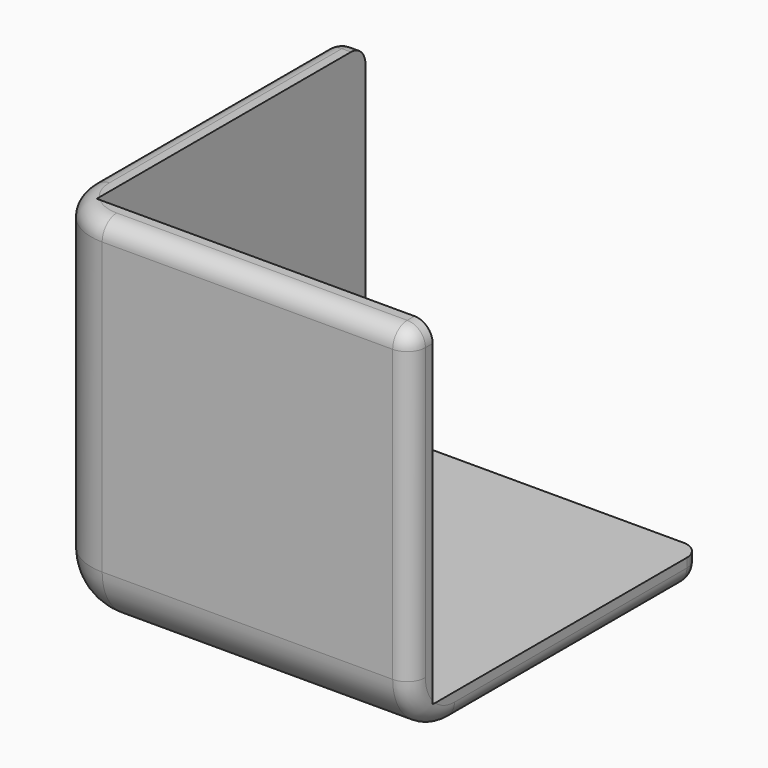
from build123d import *

# Parameters (mm, degrees)
F1_DEPTH     = 20
F3_DEPTH     = 20
F4_R         = 3
F5_T1_DEPTH  = 16
F5_T3_DEPTH  = 16
F5_T5_DEPTH  = 3
F5_T7_DEPTH  = 3
F5_T9_DEPTH  = 3
F5_T11_DEPTH = 16
F5_S15_W     = 1
F5_S15_H     = 1
F5_T16_DEPTH = 1
F5_S21_W     = 1
F5_S21_H     = 1
F5_T22_DEPTH = 1
F5_S27_W     = 1
F5_S27_H     = 1
F5_T28_DEPTH = 1
F5_T32_ANGLE = 90
F5_T34_ANGLE = 90
F5_T36_ANGLE = 90


# Not quite as in the source:
# - a fillet or chamfer that OpenCascade refuses, or shapes differently, is made with other operations: its cross-section is extruded or revolved along the edge and cut away or added


with BuildPart() as f1:
    # F0 (on Top) → F1 (new body)
    with BuildSketch(Plane.XY):
        Polygon((0, 20), (0, 0), (20, 0), (20, 1.5), (1.5, 1.5), (1.5, 20), align=None)
    extrude(amount=F1_DEPTH)

    # F2 (on Front) → F3 (join)
    with BuildSketch(Plane.XZ):
        Polygon((0, 20), (0, 0), (20, 0), (20, 1.5), (1.5, 1.5), (1.5, 20), align=None)
    extrude(amount=-F3_DEPTH)

    # F4
    f4_edges = [f1.edges().sort_by_distance(p)[0] for p in [
        (0, 0, 10),
        (0, 10, 0),
        (10, 0, 0),
    ]]
    fillet(f4_edges, radius=F4_R)

    # F5: fillet of radius 1 on 12 edges, made by hand

    # F5_s2 → F5_t1 (cut)
    with BuildSketch(Plane.XZ.offset(-19)):
        with BuildLine():
            ThreePointArc((0, 19), (0.2928932188, 19.7071067812), (1, 20))
            Line((1, 20), (0, 20))
            Line((0, 20), (0, 19))
        make_face()
        with BuildLine():
            ThreePointArc((19, 0), (19.7071067812, 0.2928932188), (20, 1))
            Line((20, 1), (20, 0))
            Line((20, 0), (19, 0))
        make_face()
    extrude(amount=F5_T1_DEPTH, mode=Mode.SUBTRACT)

    # F5_s4 → F5_t3 (cut)
    with BuildSketch(Plane.YZ.offset(3)):
        with BuildLine():
            ThreePointArc((20, 1), (19.7071067812, 0.2928932188), (19, 0))
            Line((19, 0), (20, 0))
            Line((20, 0), (20, 1))
        make_face()
        with BuildLine():
            ThreePointArc((1, 20), (0.2928932188, 19.7071067812), (0, 19))
            Line((0, 19), (0, 20))
            Line((0, 20), (1, 20))
        make_face()
    extrude(amount=F5_T3_DEPTH, mode=Mode.SUBTRACT)

    # F5_s6 → F5_t5 (cut)
    with BuildSketch(Plane.YZ.offset(1)):
        with BuildLine():
            ThreePointArc((20, 19), (19.7071067812, 19.7071067812), (19, 20))
            Line((19, 20), (20, 20))
            Line((20, 20), (20, 19))
        make_face()
    extrude(amount=F5_T5_DEPTH, mode=Mode.SUBTRACT)

    # F5_s8 → F5_t7 (cut)
    with BuildSketch(Plane.XY.offset(1)):
        with BuildLine():
            ThreePointArc((19, 20), (19.7071067812, 19.7071067812), (20, 19))
            Line((20, 19), (20, 20))
            Line((20, 20), (19, 20))
        make_face()
    extrude(amount=F5_T7_DEPTH, mode=Mode.SUBTRACT)

    # F5_s10 → F5_t9 (cut)
    with BuildSketch(Plane.XZ.offset(-4)):
        with BuildLine():
            ThreePointArc((19, 20), (19.7071067812, 19.7071067812), (20, 19))
            Line((20, 19), (20, 20))
            Line((20, 20), (19, 20))
        make_face()
    extrude(amount=F5_T9_DEPTH, mode=Mode.SUBTRACT)

    # F5_s12 → F5_t11 (cut)
    with BuildSketch(Plane.XY.offset(3)):
        with BuildLine():
            ThreePointArc((0, 19), (0.2928932188, 19.7071067812), (1, 20))
            Line((1, 20), (0, 20))
            Line((0, 20), (0, 19))
        make_face()
        with BuildLine():
            ThreePointArc((20, 1), (19.7071067812, 0.2928932188), (19, 0))
            Line((19, 0), (20, 0))
            Line((20, 0), (20, 1))
        make_face()
    extrude(amount=F5_T11_DEPTH, mode=Mode.SUBTRACT)


with BuildPart() as f5_tool14:
    # F5_s15 → F5_t16 (new body)
    with BuildSketch(Plane.YZ.offset(1)):
        with Locations((19.5, 19.5)):
            Rectangle(F5_S15_W, F5_S15_H)
    extrude(amount=-F5_T16_DEPTH)

    # F5_s17 → F5_t18 (revolve, cut)
    with BuildSketch(Plane(origin=(1, 19, 19), x_dir=(0, -0.7071067812, -0.7071067812), z_dir=(0, 0.7071067812, -0.7071067812))):
        with BuildLine():
            ThreePointArc((0, -1), (1, 0), (0, 1))
            Line((0, 1), (0, -1))
        make_face()
    revolve(axis=Axis((1, 19, 19), (-1, 0, 0)), mode=Mode.SUBTRACT)


with BuildPart() as f1_1:
    add(f1.part)

    # F5_t13: cut F5_tool14
    add(f5_tool14.part, mode=Mode.SUBTRACT)


with BuildPart() as f5_tool20:
    # F5_s21 → F5_t22 (new body)
    with BuildSketch(Plane.XZ.offset(-19)):
        with Locations((19.5, 0.5)):
            Rectangle(F5_S21_W, F5_S21_H)
    extrude(amount=-F5_T22_DEPTH)

    # F5_s23 → F5_t24 (revolve, cut)
    with BuildSketch(Plane(origin=(19, 19, 1), x_dir=(-0.7071067812, 0, 0.7071067812), z_dir=(-0.7071067812, 0, -0.7071067812))):
        with BuildLine():
            ThreePointArc((0, -1), (1, 0), (0, 1))
            Line((0, 1), (0, -1))
        make_face()
    revolve(axis=Axis((19, 19, 1), (0, 1, 0)), mode=Mode.SUBTRACT)


with BuildPart() as f1_2:
    add(f1_1.part)

    # F5_t19: cut F5_tool20
    add(f5_tool20.part, mode=Mode.SUBTRACT)


with BuildPart() as f5_tool26:
    # F5_s27 → F5_t28 (new body)
    with BuildSketch(Plane.XZ.offset(-1)):
        with Locations((19.5, 19.5)):
            Rectangle(F5_S27_W, F5_S27_H)
    extrude(amount=F5_T28_DEPTH)

    # F5_s29 → F5_t30 (revolve, cut)
    with BuildSketch(Plane(origin=(19, 1, 19), x_dir=(-0.7071067812, 0, -0.7071067812), z_dir=(-0.7071067812, 0, 0.7071067812))):
        with BuildLine():
            ThreePointArc((0, -1), (1, 0), (0, 1))
            Line((0, 1), (0, -1))
        make_face()
    revolve(axis=Axis((19, 1, 19), (0, -1, 0)), mode=Mode.SUBTRACT)


with BuildPart() as f1_3:
    add(f1_2.part)

    # F5_t25: cut F5_tool26
    add(f5_tool26.part, mode=Mode.SUBTRACT)

    # F5_s31 → F5_t32 (revolve, cut)
    with BuildSketch(Plane.XY.offset(3)):
        with BuildLine():
            ThreePointArc((1, 20), (0.2928932188, 19.7071067812), (0, 19))
            Line((0, 19), (0, 20))
            Line((0, 20), (1, 20))
        make_face()
    revolve(axis=Axis((3, 20, 3), (0, -1, 0)), revolution_arc=F5_T32_ANGLE, mode=Mode.SUBTRACT)

    # F5_s33 → F5_t34 (revolve, cut)
    with BuildSketch(Plane.XZ.offset(-3)):
        with BuildLine():
            ThreePointArc((1, 20), (0.2928932188, 19.7071067812), (0, 19))
            Line((0, 19), (0, 20))
            Line((0, 20), (1, 20))
        make_face()
    revolve(axis=Axis((3, 3, 20), (0, 0, 1)), revolution_arc=F5_T34_ANGLE, mode=Mode.SUBTRACT)

    # F5_s35 → F5_t36 (revolve, cut)
    with BuildSketch(Plane.XZ.offset(-3)):
        with BuildLine():
            ThreePointArc((20, 1), (19.7071067812, 0.2928932188), (19, 0))
            Line((19, 0), (20, 0))
            Line((20, 0), (20, 1))
        make_face()
    revolve(axis=Axis((20, 3, 3), (-1, 0, 0)), revolution_arc=F5_T36_ANGLE, mode=Mode.SUBTRACT)


solid = f1_3.part
